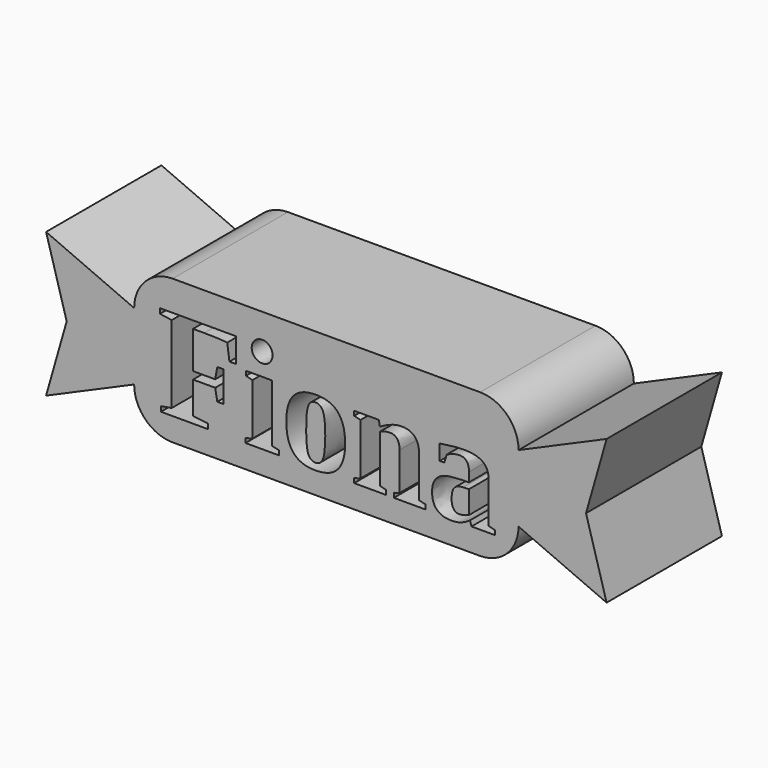
from build123d import *

# Parameters (mm, degrees)
F1_DEPTH     = 19.05
F2_TEXT_SIZE = 18.3464794031
F3_DEPTH     = 35.052


# Not quite as in the source:
# - Text() gives the source's letters only with a copy of the font that has no kerning and outlines rounded to 1/6400 em; it was checked with that copy


with BuildPart() as f1:
    # F0 (on Front) → F1 (new body)
    with BuildSketch(Plane.XZ):
        with BuildLine():
            Line((14.0663449314, 7.925544067), (-26.5736550686, 7.925544067))
            ThreePointArc((-26.5736550686, 7.925544067), (-30.165757517, 6.4376465154), (-31.6536550686, 2.845544067))
            Line((-31.6536550686, 2.845544067), (-31.6536550686, -6.044455933))
            ThreePointArc((-31.6536550686, -6.044455933), (-30.165757517, -9.6365583815), (-26.5736550686, -11.124455933))
            Line((-26.5736550686, -11.124455933), (14.0663449314, -11.124455933))
            ThreePointArc((14.0663449314, -11.124455933), (17.6584473799, -9.6365583815), (19.1463449314, -6.044455933))
            Line((19.1463449314, -6.044455933), (19.1463449314, 2.845544067))
            ThreePointArc((19.1463449314, 2.845544067), (17.6584473799, 6.4376465154), (14.0663449314, 7.925544067))
        make_face()
        Polygon((-31.6536550686, -6.044455933), (-31.6536550686, 2.845544067), (-43.2933973338, 7.925544067), (-40.5725131025, -1.599455933), (-43.2933973338, -11.124455933), align=None)
        Polygon((30.7860871966, 7.925544067), (19.1463449314, 2.845544067), (19.1463449314, -6.044455933), (30.7860871966, -11.124455933), (28.0652029653, -1.599455933), align=None)
    extrude(amount=F1_DEPTH)

    # F2 (on face) → F3 (cut)
    with BuildSketch(Plane.XZ.offset(19.05)):
        with Locations((-28.5476521574, -8.0665309992)):
            Text('Fiona', F2_TEXT_SIZE, font='Tinos', font_style=FontStyle.BOLD, text_align=(TextAlign.LEFT, TextAlign.BOTTOM))
    extrude(amount=-F3_DEPTH, mode=Mode.SUBTRACT)


solid = f1.part
